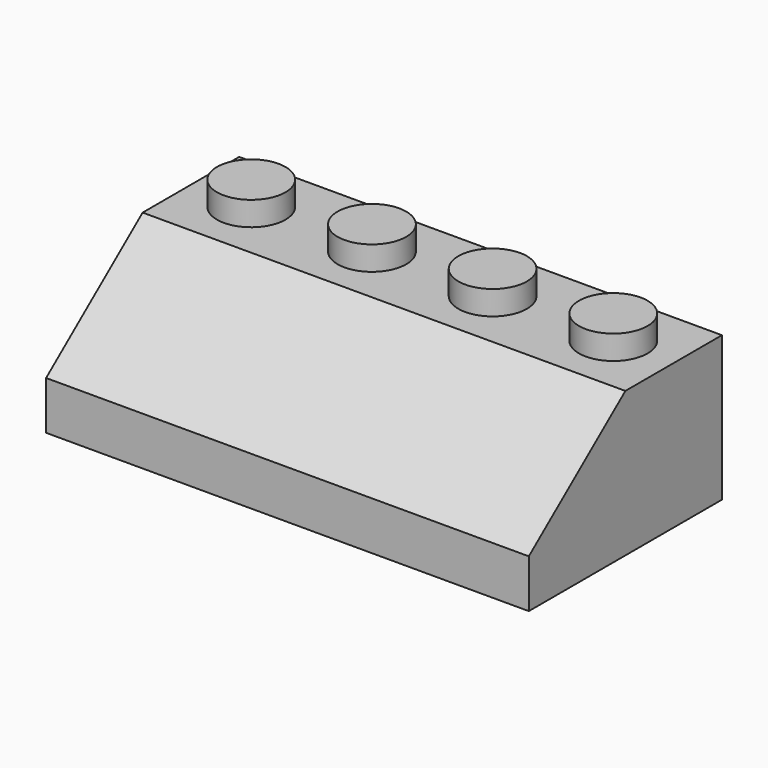
from build123d import *

# Parameters (mm, degrees)
F0_W     = 31.75
F0_H     = 15.875
F0_R     = 2.2550277878
F1_DEPTH = 9.525
F2_DEPTH = 11.1125
F4_DEPTH = 31.751
F5_T     = -1.5875


# Not quite as in the source:
# - a feature names something its author has since deleted; it is built from what else it names


with BuildPart() as f1:
    # F0 (on Top) → F1 (new body)
    with BuildSketch(Plane.XY):
        Rectangle(F0_W, F0_H)
        with Locations((-11.90625, 3.96875)):
            Circle(F0_R, mode=Mode.SUBTRACT)
        with Locations((-3.96875, 3.96875)):
            Circle(F0_R, mode=Mode.SUBTRACT)
        with Locations((3.96875, 3.96875)):
            Circle(F0_R, mode=Mode.SUBTRACT)
        with Locations((11.90625, 3.96875)):
            Circle(F0_R, mode=Mode.SUBTRACT)
    extrude(amount=F1_DEPTH)

    # F0 (on Top) → F2 (join)
    with BuildSketch(Plane.XY):
        with Locations((-11.90625, 3.96875)):
            Circle(F0_R)
        with Locations((-3.96875, 3.96875)):
            Circle(F0_R)
        with Locations((3.96875, 3.96875)):
            Circle(F0_R)
        with Locations((11.90625, 3.96875)):
            Circle(F0_R)
    extrude(amount=F2_DEPTH)

    # F3 (on face) → F4 (cut, through all)
    with BuildSketch(Plane.YZ.offset(15.875)):
        Polygon((-7.9375, 9.525), (-7.9375, 3.175), (0, 9.525), align=None)
    extrude(amount=-F4_DEPTH, mode=Mode.SUBTRACT)

    # F5
    f5_openings = [f1.faces().sort_by_distance(p)[0] for p in [
        (0, 0, 0),
    ]]
    offset(amount=F5_T, openings=f5_openings, kind=Kind.INTERSECTION)


solid = f1.part
